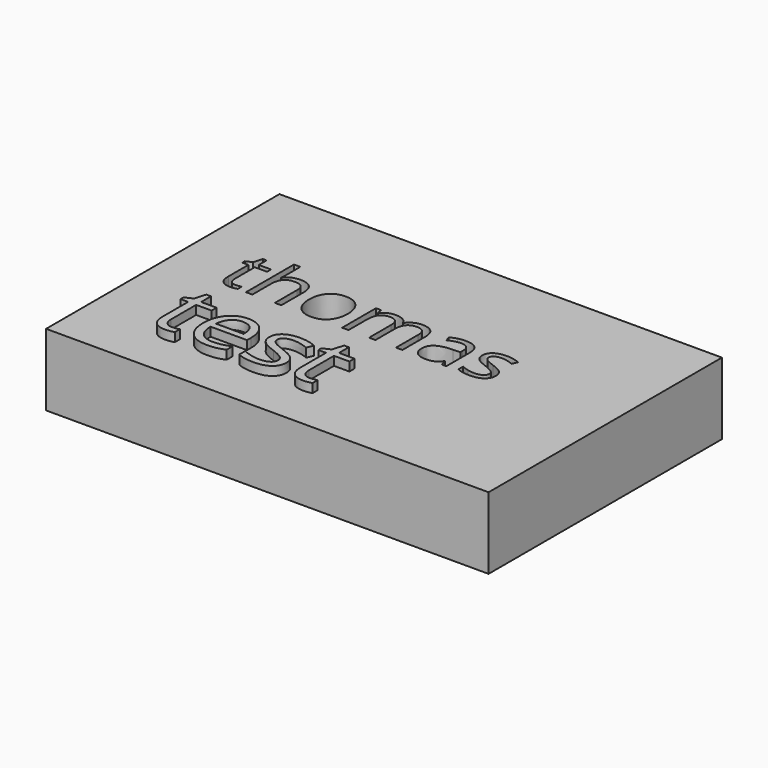
from build123d import *

# Parameters (mm, degrees)
F0_W         = 199.5291560888
F0_H         = 131.5212398767
F1_DEPTH     = 32.4
F2_TEXT_SIZE = 44.6849644908
F3_DEPTH     = 4


# Not quite as in the source:
# - Text() gives the source's letters only with a copy of the font that has no kerning and outlines rounded to 1/6400 em; it was checked with that copy


with BuildPart() as f1:
    # F0 (on Top) → F1 (new body)
    with BuildSketch(Plane.XY):
        Rectangle(F0_W, F0_H)
        with BuildLine():
            add(Edge.make_bspline(
                [(-70.8970974245, 2.9569819631), (-70.0792679822, 2.0362284073), (-68.6550207902, 2.0362284073)],
                knots=[0, 0, 0, 1, 1, 1], degree=2))
            add(Edge.make_bspline(
                [(-68.6550207902, 2.0362284073), (-67.8872625382, 2.0362284073), (-67.1751389422, 2.1474977192)],
                knots=[0, 0, 0, 1, 1, 1], degree=2))
            add(Edge.make_bspline(
                [(-67.1751389422, 2.1474977192), (-66.4630153462, 2.2587670311), (-66.0457554267, 2.3811632741)],
                knots=[0, 0, 0, 1, 1, 1], degree=2))
            Line((-66.0457554267, 2.3811632741), (-66.0457554267, 0.1724674334))
            add(Edge.make_bspline(
                [(-66.0457554267, 0.1724674334), (-66.5130865366, -0.0500711903), (-67.4254948939, -0.2002847614)],
                knots=[0, 0, 0, 1, 1, 1], degree=2))
            add(Edge.make_bspline(
                [(-67.4254948939, -0.2002847614), (-68.3379032513, -0.3504983324), (-69.0722807097, -0.3504983324)],
                knots=[0, 0, 0, 1, 1, 1], degree=2))
            add(Edge.make_bspline(
                [(-69.0722807097, -0.3504983324), (-74.5968020443, -0.3504983324), (-74.5968020443, 5.4744501443)],
                knots=[0, 0, 0, 1, 1, 1], degree=2))
            Line((-74.5968020443, 5.4744501443), (-74.5968020443, 16.8127930245))
            Line((-74.5968020443, 16.8127930245), (-77.3284636509, 16.8127930245))
            Line((-77.3284636509, 16.8127930245), (-77.3284636509, 18.2036594229))
            Line((-77.3284636509, 18.2036594229), (-74.5968020443, 19.4053679912))
            Line((-74.5968020443, 19.4053679912), (-73.3839665449, 23.4722613402))
            Line((-73.3839665449, 23.4722613402), (-71.7149268668, 23.4722613402))
            Line((-71.7149268668, 23.4722613402), (-71.7149268668, 19.0548696588))
            Line((-71.7149268668, 19.0548696588), (-66.1848420665, 19.0548696588))
            Line((-66.1848420665, 19.0548696588), (-66.1848420665, 16.8127930245))
            Line((-66.1848420665, 16.8127930245), (-71.7149268668, 16.8127930245))
            Line((-71.7149268668, 16.8127930245), (-71.7149268668, 5.5968463874))
            add(Edge.make_bspline(
                [(-71.7149268668, 5.5968463874), (-71.7149268668, 3.8777355189), (-70.8970974245, 2.9569819631)],
                knots=[0, 0, 0, 1, 1, 1], degree=2))
        make_face(mode=Mode.SUBTRACT)
        with BuildLine():
            Line((-46.3121429655, 0), (-49.1995816087, 0))
            Line((-49.1995816087, 0), (-49.1995816087, 12.3286397559))
            add(Edge.make_bspline(
                [(-49.1995816087, 12.3286397559), (-49.1995816087, 14.6541683741), (-50.2594218043, 15.8030240192)],
                knots=[0, 0, 0, 1, 1, 1], degree=2))
            add(Edge.make_bspline(
                [(-50.2594218043, 15.8030240192), (-51.3192619999, 16.9518796643), (-53.5835924966, 16.9518796643)],
                knots=[0, 0, 0, 1, 1, 1], degree=2))
            add(Edge.make_bspline(
                [(-53.5835924966, 16.9518796643), (-56.5878639172, 16.9518796643), (-57.9703851173, 15.3162207797)],
                knots=[0, 0, 0, 1, 1, 1], degree=2))
            add(Edge.make_bspline(
                [(-57.9703851173, 15.3162207797), (-59.3529063173, 13.6805618951), (-59.3529063173, 9.9641668785)],
                knots=[0, 0, 0, 1, 1, 1], degree=2))
            Line((-59.3529063173, 9.9641668785), (-59.3529063173, 0))
            Line((-59.3529063173, 0), (-62.2403449605, 0))
            Line((-62.2403449605, 0), (-62.2403449605, 27.0551331826))
            Line((-62.2403449605, 27.0551331826), (-59.3529063173, 27.0551331826))
            Line((-59.3529063173, 27.0551331826), (-59.3529063173, 18.8657118286))
            add(Edge.make_bspline(
                [(-59.3529063173, 18.8657118286), (-59.3529063173, 17.3858299806), (-59.4919929572, 16.4122235017)],
                knots=[0, 0, 0, 1, 1, 1], degree=2))
            Line((-59.4919929572, 16.4122235017), (-59.3195255238, 16.4122235017))
            add(Edge.make_bspline(
                [(-59.3195255238, 16.4122235017), (-58.4683152879, 17.7863995034), (-56.8938545249, 18.5764116177)],
                knots=[0, 0, 0, 1, 1, 1], degree=2))
            add(Edge.make_bspline(
                [(-56.8938545249, 18.5764116177), (-55.3193937618, 19.366423732), (-53.3054192169, 19.366423732)],
                knots=[0, 0, 0, 1, 1, 1], degree=2))
            add(Edge.make_bspline(
                [(-53.3054192169, 19.366423732), (-49.811562824, 19.366423732), (-48.0618528947, 17.7057292523)],
                knots=[0, 0, 0, 1, 1, 1], degree=2))
            add(Edge.make_bspline(
                [(-48.0618528947, 17.7057292523), (-46.3121429655, 16.0450347725), (-46.3121429655, 12.4287821365)],
                knots=[0, 0, 0, 1, 1, 1], degree=2))
            Line((-46.3121429655, 12.4287821365), (-46.3121429655, 0))
        make_face(mode=Mode.SUBTRACT)
        with BuildLine():
            add(Edge.make_bspline(
                [(-26.2975754918, 16.7432497045), (-23.9414478128, 14.0811314179), (-23.9414478128, 9.546906959)],
                knots=[0, 0, 0, 1, 1, 1], degree=2))
            add(Edge.make_bspline(
                [(-23.9414478128, 9.546906959), (-23.9414478128, 4.8847227914), (-26.2864485606, 2.2671122295)],
                knots=[0, 0, 0, 1, 1, 1], degree=2))
            add(Edge.make_bspline(
                [(-26.2864485606, 2.2671122295), (-28.6314493084, -0.3504983324), (-32.7706677102, -0.3504983324)],
                knots=[0, 0, 0, 1, 1, 1], degree=2))
            add(Edge.make_bspline(
                [(-32.7706677102, -0.3504983324), (-35.3298618833, -0.3504983324), (-37.3104556347, 0.8512102359)],
                knots=[0, 0, 0, 1, 1, 1], degree=2))
            add(Edge.make_bspline(
                [(-37.3104556347, 0.8512102359), (-39.2910493861, 2.0529188041), (-40.3703617113, 4.2949954384)],
                knots=[0, 0, 0, 1, 1, 1], degree=2))
            add(Edge.make_bspline(
                [(-40.3703617113, 4.2949954384), (-41.4496740365, 6.5370720727), (-41.4496740365, 9.546906959)],
                knots=[0, 0, 0, 1, 1, 1], degree=2))
            add(Edge.make_bspline(
                [(-41.4496740365, 9.546906959), (-41.4496740365, 14.203527661), (-39.1185819527, 16.8044478261)],
                knots=[0, 0, 0, 1, 1, 1], degree=2))
            add(Edge.make_bspline(
                [(-39.1185819527, 16.8044478261), (-36.7874898689, 19.4053679912), (-32.6482714671, 19.4053679912)],
                knots=[0, 0, 0, 1, 1, 1], degree=2))
            add(Edge.make_bspline(
                [(-32.6482714671, 19.4053679912), (-28.6537031708, 19.4053679912), (-26.2975754918, 16.7432497045)],
                knots=[0, 0, 0, 1, 1, 1], degree=2))
        make_face(mode=Mode.SUBTRACT)
        with BuildLine():
            Line((8.2932718376, 0), (5.41139666, 0))
            Line((5.41139666, 0), (5.41139666, 12.395401343))
            add(Edge.make_bspline(
                [(5.41139666, 12.395401343), (5.41139666, 14.6764222364), (4.4377901811, 15.8141509504)],
                knots=[0, 0, 0, 1, 1, 1], degree=2))
            add(Edge.make_bspline(
                [(4.4377901811, 15.8141509504), (3.4641837022, 16.9518796643), (1.4112648981, 16.9518796643)],
                knots=[0, 0, 0, 1, 1, 1], degree=2))
            add(Edge.make_bspline(
                [(1.4112648981, 16.9518796643), (-1.2814524493, 16.9518796643), (-2.5693947343, 15.4052362292)],
                knots=[0, 0, 0, 1, 1, 1], degree=2))
            add(Edge.make_bspline(
                [(-2.5693947343, 15.4052362292), (-3.8573370192, 13.8585927941), (-3.8573370192, 10.6429096809)],
                knots=[0, 0, 0, 1, 1, 1], degree=2))
            Line((-3.8573370192, 10.6429096809), (-3.8573370192, 0))
            Line((-3.8573370192, 0), (-6.7447756624, 0))
            Line((-6.7447756624, 0), (-6.7447756624, 12.395401343))
            add(Edge.make_bspline(
                [(-6.7447756624, 12.395401343), (-6.7447756624, 14.6764222364), (-7.7183821413, 15.8141509504)],
                knots=[0, 0, 0, 1, 1, 1], degree=2))
            add(Edge.make_bspline(
                [(-7.7183821413, 15.8141509504), (-8.6919886202, 16.9518796643), (-10.7615978211, 16.9518796643)],
                knots=[0, 0, 0, 1, 1, 1], degree=2))
            add(Edge.make_bspline(
                [(-10.7615978211, 16.9518796643), (-13.4710055653, 16.9518796643), (-14.7311305223, 15.3273477109)],
                knots=[0, 0, 0, 1, 1, 1], degree=2))
            add(Edge.make_bspline(
                [(-14.7311305223, 15.3273477109), (-15.9912554793, 13.7028157575), (-15.9912554793, 9.9975476721)],
                knots=[0, 0, 0, 1, 1, 1], degree=2))
            Line((-15.9912554793, 9.9975476721), (-15.9912554793, 0))
            Line((-15.9912554793, 0), (-18.8786941225, 0))
            Line((-18.8786941225, 0), (-18.8786941225, 19.0548696588))
            Line((-18.8786941225, 19.0548696588), (-16.5309116419, 19.0548696588))
            Line((-16.5309116419, 19.0548696588), (-16.063580532, 16.4456042953))
            Line((-16.063580532, 16.4456042953), (-15.9244938922, 16.4456042953))
            add(Edge.make_bspline(
                [(-15.9244938922, 16.4456042953), (-15.1066644499, 17.8364706937), (-13.6184374035, 18.6209193424)],
                knots=[0, 0, 0, 1, 1, 1], degree=2))
            add(Edge.make_bspline(
                [(-13.6184374035, 18.6209193424), (-12.1302103572, 19.4053679912), (-10.2887032457, 19.4053679912)],
                knots=[0, 0, 0, 1, 1, 1], degree=2))
            add(Edge.make_bspline(
                [(-10.2887032457, 19.4053679912), (-5.8212403738, 19.4053679912), (-4.4470643722, 16.1674310156)],
                knots=[0, 0, 0, 1, 1, 1], degree=2))
            Line((-4.4470643722, 16.1674310156), (-4.3079777323, 16.1674310156))
            add(Edge.make_bspline(
                [(-4.3079777323, 16.1674310156), (-3.4567674965, 17.6640032603), (-1.8405807415, 18.5346856257)],
                knots=[0, 0, 0, 1, 1, 1], degree=2))
            add(Edge.make_bspline(
                [(-1.8405807415, 18.5346856257), (-0.2243939865, 19.4053679912), (1.8452152144, 19.4053679912)],
                knots=[0, 0, 0, 1, 1, 1], degree=2))
            add(Edge.make_bspline(
                [(1.8452152144, 19.4053679912), (5.0775887244, 19.4053679912), (6.685430281, 17.7446735114)],
                knots=[0, 0, 0, 1, 1, 1], degree=2))
            add(Edge.make_bspline(
                [(6.685430281, 17.7446735114), (8.2932718376, 16.0839790317), (8.2932718376, 12.4287821365)],
                knots=[0, 0, 0, 1, 1, 1], degree=2))
            Line((8.2932718376, 12.4287821365), (8.2932718376, 0))
        make_face(mode=Mode.SUBTRACT)
        with BuildLine():
            Line((28.0992093515, 0), (25.9572750979, 0))
            Line((25.9572750979, 0), (25.3842381418, 2.7149712098))
            Line((25.3842381418, 2.7149712098), (25.2451515019, 2.7149712098))
            add(Edge.make_bspline(
                [(25.2451515019, 2.7149712098), (23.8209043099, 0.9235352886), (22.4050023163, 0.2865184781)],
                knots=[0, 0, 0, 1, 1, 1], degree=2))
            add(Edge.make_bspline(
                [(22.4050023163, 0.2865184781), (20.9891003227, -0.3504983324), (18.8638564658, -0.3504983324)],
                knots=[0, 0, 0, 1, 1, 1], degree=2))
            add(Edge.make_bspline(
                [(18.8638564658, -0.3504983324), (16.0320524786, -0.3504983324), (14.424210922, 1.1126931188)],
                knots=[0, 0, 0, 1, 1, 1], degree=2))
            add(Edge.make_bspline(
                [(14.424210922, 1.1126931188), (12.8163693654, 2.5758845699), (12.8163693654, 5.2686019173)],
                knots=[0, 0, 0, 1, 1, 1], degree=2))
            add(Edge.make_bspline(
                [(12.8163693654, 5.2686019173), (12.8163693654, 11.0379157381), (22.0461587855, 11.3160890178)],
                knots=[0, 0, 0, 1, 1, 1], degree=2))
            Line((22.0461587855, 11.3160890178), (25.2785322955, 11.4217948641))
            Line((25.2785322955, 11.4217948641), (25.2785322955, 12.6068130355))
            add(Edge.make_bspline(
                [(25.2785322955, 12.6068130355), (25.2785322955, 14.8488896698), (24.3160527478, 15.9170750639)],
                knots=[0, 0, 0, 1, 1, 1], degree=2))
            add(Edge.make_bspline(
                [(24.3160527478, 15.9170750639), (23.3535732, 16.9852604579), (21.2283293432, 16.9852604579)],
                knots=[0, 0, 0, 1, 1, 1], degree=2))
            add(Edge.make_bspline(
                [(21.2283293432, 16.9852604579), (18.8471660691, 16.9852604579), (15.8428946484, 15.5276324723)],
                knots=[0, 0, 0, 1, 1, 1], degree=2))
            Line((15.8428946484, 15.5276324723), (14.9527401534, 17.736328313))
            add(Edge.make_bspline(
                [(14.9527401534, 17.736328313), (16.3602969486, 18.4985230994), (18.0376818252, 18.9324734157)],
                knots=[0, 0, 0, 1, 1, 1], degree=2))
            add(Edge.make_bspline(
                [(18.0376818252, 18.9324734157), (19.7150667017, 19.366423732), (21.4063602422, 19.366423732)],
                knots=[0, 0, 0, 1, 1, 1], degree=2))
            add(Edge.make_bspline(
                [(21.4063602422, 19.366423732), (24.8112011856, 19.366423732), (26.4552052686, 17.8559428233)],
                knots=[0, 0, 0, 1, 1, 1], degree=2))
            add(Edge.make_bspline(
                [(26.4552052686, 17.8559428233), (28.0992093515, 16.3454619146), (28.0992093515, 13.0073825583)],
                knots=[0, 0, 0, 1, 1, 1], degree=2))
            Line((28.0992093515, 13.0073825583), (28.0992093515, 0))
        make_face(mode=Mode.SUBTRACT)
        with BuildLine():
            add(Edge.make_bspline(
                [(45.1401044653, 8.3451983907), (46.3306861024, 7.0934186321), (46.3306861024, 5.1962768646)],
                knots=[0, 0, 0, 1, 1, 1], degree=2))
            add(Edge.make_bspline(
                [(46.3306861024, 5.1962768646), (46.3306861024, 2.5369403108), (44.350092351, 1.0932209892)],
                knots=[0, 0, 0, 1, 1, 1], degree=2))
            add(Edge.make_bspline(
                [(44.350092351, 1.0932209892), (42.3694985996, -0.3504983324), (38.7866267572, -0.3504983324)],
                knots=[0, 0, 0, 1, 1, 1], degree=2))
            add(Edge.make_bspline(
                [(38.7866267572, -0.3504983324), (34.9979066879, -0.3504983324), (32.8782262966, 0.8512102359)],
                knots=[0, 0, 0, 1, 1, 1], degree=2))
            Line((32.8782262966, 0.8512102359), (32.8782262966, 3.5272371865))
            add(Edge.make_bspline(
                [(32.8782262966, 3.5272371865), (34.2524022983, 2.8318039872), (35.8240813285, 2.4340161973)],
                knots=[0, 0, 0, 1, 1, 1], degree=2))
            add(Edge.make_bspline(
                [(35.8240813285, 2.4340161973), (37.3957603588, 2.0362284073), (38.8589518099, 2.0362284073)],
                knots=[0, 0, 0, 1, 1, 1], degree=2))
            add(Edge.make_bspline(
                [(38.8589518099, 2.0362284073), (41.117718841, 2.0362284073), (42.3333360733, 2.7566972017)],
                knots=[0, 0, 0, 1, 1, 1], degree=2))
            add(Edge.make_bspline(
                [(42.3333360733, 2.7566972017), (43.5489533055, 3.4771659961), (43.5489533055, 4.9570478441)],
                knots=[0, 0, 0, 1, 1, 1], degree=2))
            add(Edge.make_bspline(
                [(43.5489533055, 4.9570478441), (43.5489533055, 6.0697409628), (42.5864737578, 6.8597530772)],
                knots=[0, 0, 0, 1, 1, 1], degree=2))
            add(Edge.make_bspline(
                [(42.5864737578, 6.8597530772), (41.6239942101, 7.6497651915), (38.8200075508, 8.7290775167)],
                knots=[0, 0, 0, 1, 1, 1], degree=2))
            add(Edge.make_bspline(
                [(38.8200075508, 8.7290775167), (36.160670997, 9.7193743924), (35.0396326798, 10.4593153163)],
                knots=[0, 0, 0, 1, 1, 1], degree=2))
            add(Edge.make_bspline(
                [(35.0396326798, 10.4593153163), (33.9185943627, 11.1992562403), (33.3705930017, 12.1367001929)],
                knots=[0, 0, 0, 1, 1, 1], degree=2))
            add(Edge.make_bspline(
                [(33.3705930017, 12.1367001929), (32.8225916407, 13.0741441454), (32.8225916407, 14.3759950944)],
                knots=[0, 0, 0, 1, 1, 1], degree=2))
            add(Edge.make_bspline(
                [(32.8225916407, 14.3759950944), (32.8225916407, 16.7070871782), (34.7197334082, 18.0562275847)],
                knots=[0, 0, 0, 1, 1, 1], degree=2))
            add(Edge.make_bspline(
                [(34.7197334082, 18.0562275847), (36.6168751756, 19.4053679912), (39.9160102728, 19.4053679912)],
                knots=[0, 0, 0, 1, 1, 1], degree=2))
            add(Edge.make_bspline(
                [(39.9160102728, 19.4053679912), (42.9926067461, 19.4053679912), (45.9356800453, 18.1535882326)],
                knots=[0, 0, 0, 1, 1, 1], degree=2))
            Line((45.9356800453, 18.1535882326), (44.9064389104, 15.805805752))
            add(Edge.make_bspline(
                [(44.9064389104, 15.805805752), (42.0412541296, 16.9852604579), (39.7101620458, 16.9852604579)],
                knots=[0, 0, 0, 1, 1, 1], degree=2))
            add(Edge.make_bspline(
                [(39.7101620458, 16.9852604579), (37.6572432417, 16.9852604579), (36.6140934428, 16.3426801818)],
                knots=[0, 0, 0, 1, 1, 1], degree=2))
            add(Edge.make_bspline(
                [(36.6140934428, 16.3426801818), (35.570943644, 15.7000999057), (35.570943644, 14.5707163902)],
                knots=[0, 0, 0, 1, 1, 1], degree=2))
            add(Edge.make_bspline(
                [(35.570943644, 14.5707163902), (35.570943644, 13.8029581382), (35.9631679684, 13.2660837084)],
                knots=[0, 0, 0, 1, 1, 1], degree=2))
            add(Edge.make_bspline(
                [(35.9631679684, 13.2660837084), (36.3553922927, 12.7292092786), (37.2232929254, 12.2424060391)],
                knots=[0, 0, 0, 1, 1, 1], degree=2))
            add(Edge.make_bspline(
                [(37.2232929254, 12.2424060391), (38.091193558, 11.7556027997), (40.5613722816, 10.8320675111)],
                knots=[0, 0, 0, 1, 1, 1], degree=2))
            add(Edge.make_bspline(
                [(40.5613722816, 10.8320675111), (43.9495228283, 9.5969781493), (45.1401044653, 8.3451983907)],
                knots=[0, 0, 0, 1, 1, 1], degree=2))
        make_face(mode=Mode.SUBTRACT)
    extrude(amount=F1_DEPTH)

    # F2 (on face) → F3 (join)
    with BuildSketch(Plane.XY.offset(32.4)):
        with Locations((-72.8329643607, -45.5997735262)):
            Text('test', F2_TEXT_SIZE, font='Open Sans', text_align=(TextAlign.LEFT, TextAlign.BOTTOM))
    extrude(amount=F3_DEPTH)


solid = f1.part
